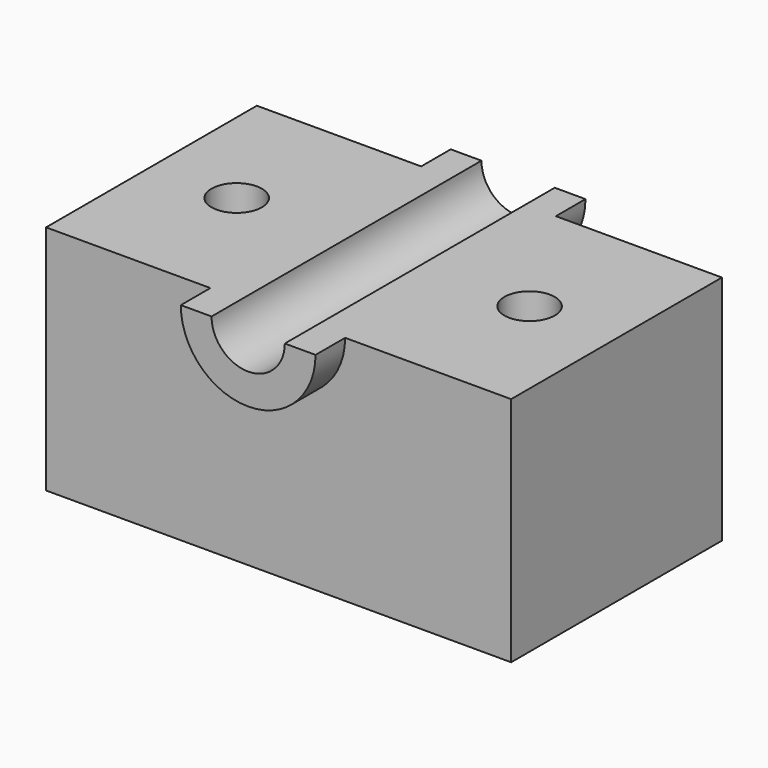
from build123d import *

# Parameters (mm, degrees)
F1_DEPTH = 43.434
F2_DEPTH = 55.626
F3_R     = 8.3189115378
F4_DEPTH = 76.3916911016


# Not quite as in the source:
# - a pattern or mirror of a feature is missing from the dataset's text; its kind, count and spacing are read off the source's solid


with BuildPart() as f1:
    # F0 (on Front) → F1 (new body, symmetric)
    with BuildSketch(Plane.XZ):
        with BuildLine():
            ThreePointArc((22.2132560443, 0), (0, -22.2132560443), (-22.2132560443, 0))
            Line((-22.2132560443, 0), (-76.3906985521, 0))
            Line((-76.3906985521, 0), (-76.3906985521, -76.3906911016))
            Line((-76.3906985521, -76.3906911016), (76.9618302584, -76.3906911016))
            Line((76.9618302584, -76.3906911016), (76.9618302584, 0))
            Line((76.9618302584, 0), (22.2132560443, 0))
        make_face()
    extrude(amount=F1_DEPTH, both=True)

    # F0 (on Front) → F2 (join, symmetric)
    with BuildSketch(Plane.XZ):
        with BuildLine():
            ThreePointArc((12.0770555024, 0), (0, -12.0770555024), (-12.0770555024, 0))
            Line((-12.0770555024, 0), (-22.2132560443, 0))
            ThreePointArc((-22.2132560443, 0), (0, -22.2132560443), (22.2132560443, 0))
            Line((22.2132560443, 0), (12.0770555024, 0))
        make_face()
    extrude(amount=F2_DEPTH, both=True)

    # F3 (on face) → F4 (cut, through all)
    with BuildSketch(Plane.XY):
        with Locations((48.2908003032, 0)):
            Circle(F3_R)
    f4 = extrude(amount=-F4_DEPTH, mode=Mode.SUBTRACT)

    # F4_copies: F4 across plane
    add(f4.mirror(Plane(origin=(0, 0, 0), x_dir=(0, 0, -1), z_dir=(-1, 0, 0))), mode=Mode.SUBTRACT)


solid = f1.part
